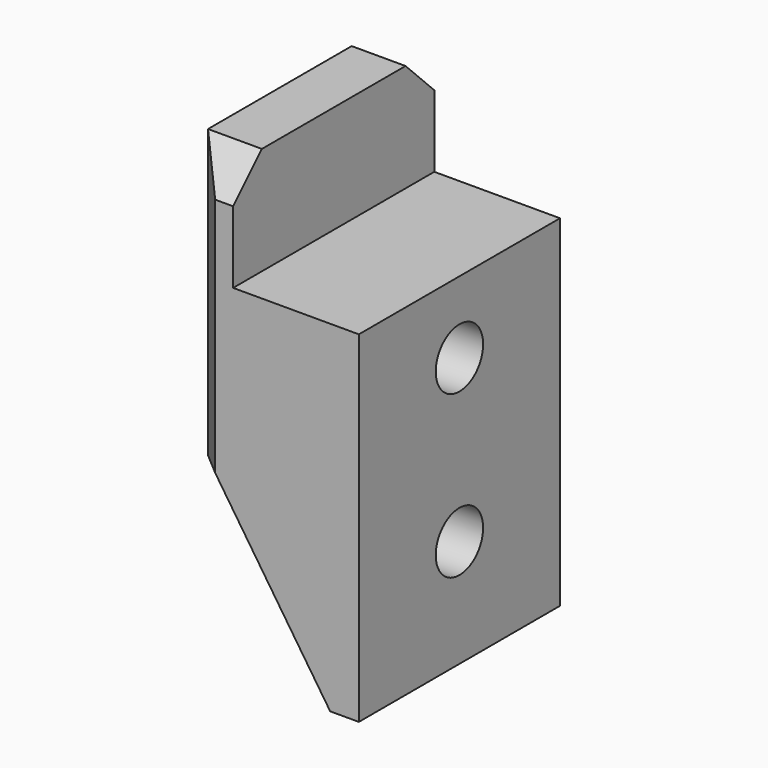
from build123d import *

# Parameters (mm, degrees)
F1_DEPTH       = 7
F2_R           = 3.5
F3_DEPTH       = 4
F4_D           = 3.3
F4_START       = 4
F4_START_2     = 4.24
F4_CSINK_D     = 6.72
F4_CSINK_ANGLE = 90
F5_T1_DEPTH    = 20.2867319519
F5_T3_DEPTH    = 26.2867319519
F5_T5_DEPTH    = 21.1033857783
F5_T7_DEPTH    = 19.707629012
F6_W           = 7
F6_H           = 6
F7_DEPTH       = 7.001
F7_DEPTH_BACK  = 7.001


# Not quite as in the source:
# - a fillet or chamfer that OpenCascade refuses, or shapes differently, is made with other operations: its cross-section is extruded or revolved along the edge and cut away or added


with BuildPart() as f1:
    # F0 (on Front) → F1 (new body, symmetric)
    with BuildSketch(Plane.XZ):
        Polygon((0, -25), (0, 0), (-10, 0), (-10, -16), (-4, -25), align=None)
    extrude(amount=F1_DEPTH, both=True)

    # F2 (on face) → F3 (cut)
    with BuildSketch(Plane(origin=(-10, 0, 0), x_dir=(0, -1, 0), z_dir=(-1, 0, 0))):
        with Locations((0, -10)):
            Circle(F2_R)
        with Locations((0, -19)):
            Circle(F2_R)
    extrude(amount=-F3_DEPTH, mode=Mode.SUBTRACT)

    # F4 (through all)
    # its depths count from where the whole tool has entered the part; down to there all is cleared
    with Locations(Plane(origin=(-10, 0, 0), x_dir=(0, -1, 0), z_dir=(-1, 0, 0))):
        with Locations((0, -19, -F4_START_2), (0, -10, -F4_START)):
            CounterSinkHole(F4_D / 2, F4_CSINK_D / 2, counter_sink_angle=F4_CSINK_ANGLE)

    # F5: chamfer of 2 on 7 edges, made by hand

    # F5_s2 → F5_t1 (cut)
    with BuildSketch(Plane.YZ.offset(-15.1433659759)):
        Polygon((-7, -2), (-5, 0), (-7, 0), align=None)
        Polygon((7, -2), (5, 0), (7, 0), align=None)
    extrude(amount=F5_T1_DEPTH, mode=Mode.SUBTRACT)

    # F5_s4 → F5_t3 (cut)
    with BuildSketch(Plane.XY.offset(-21.1433659759)):
        Polygon((-8, 7), (-10, 5), (-10, 7), align=None)
        Polygon((-8, -7), (-10, -5), (-10, -7), align=None)
    extrude(amount=F5_T3_DEPTH, mode=Mode.SUBTRACT)

    # F5_s6 → F5_t5 (cut)
    with BuildSketch(Plane(origin=(1.4546661916, 0, -2.1819992874), x_dir=(0, 1, 0), z_dir=(0.5547001962, 0, -0.8320502943))):
        Polygon((-7, -15.195706083), (-5, -17.195706083), (-7, -17.195706083), align=None)
        Polygon((7, -15.195706083), (5, -17.195706083), (7, -17.195706083), align=None)
    extrude(amount=F5_T5_DEPTH, mode=Mode.SUBTRACT)

    # F5_s8 → F5_t7 (cut)
    with BuildSketch(Plane.XZ.offset(-9.853814506)):
        Polygon((-2.929632483, -25), (-4.5937330717, -24.1094003925), (-4, -25), align=None)
    extrude(amount=F5_T7_DEPTH, mode=Mode.SUBTRACT)

    # F6 (on Front) → F7 (cut, two sides)
    with BuildSketch(Plane.XZ) as f7_sk:
        with Locations((-3.5, -3)):
            Rectangle(F6_W, F6_H)
    extrude(amount=-F7_DEPTH, mode=Mode.SUBTRACT)
    extrude(f7_sk.sketch, amount=F7_DEPTH_BACK, mode=Mode.SUBTRACT)


solid = f1.part
